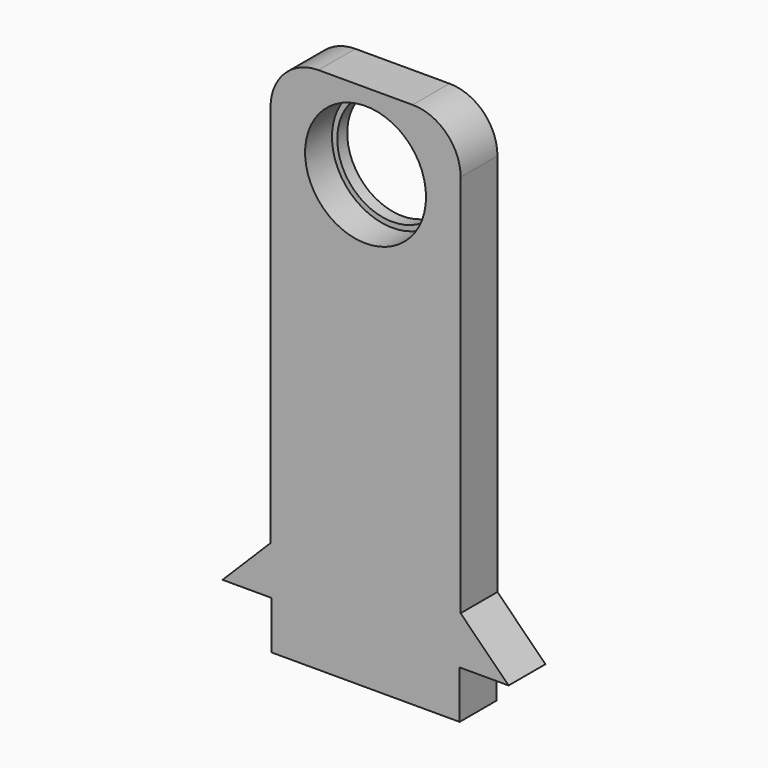
from build123d import *

# Parameters (mm, degrees)
F0_W      = 19.8
F0_H      = 55
F1_DEPTH  = 4.8
F2_R      = 5.75
F3_DEPTH  = 4.8
F4_R      = 6.3
F5_DEPTH  = 3.5
F6_W      = 4.8
F6_H      = 5
F7_DEPTH  = 5
F8_SIZE   = 4.99999
F9_W      = 4.8
F9_H      = 5
F10_DEPTH = 5
F11_SIZE  = 4.99999
F12_R     = 5
F13_DEPTH = 0.1
F14_DEPTH = 0.1


# Not quite as in the source:
# - a fillet or chamfer is up to 0.001 mm smaller than in the source, because OpenCascade refuses the exact size


with BuildPart() as f1:
    # F0 (on Front) → F1 (new body)
    with BuildSketch(Plane.XZ):
        with Locations((-0.9316042997, 16.8101646874)):
            Rectangle(F0_W, F0_H)
    extrude(amount=F1_DEPTH)

    # F2 (on face) → F3 (cut, through all)
    with BuildSketch(Plane.XZ.offset(4.8)):
        with Locations((-0.9316042997, 36.3101646874)):
            Circle(F2_R)
    extrude(amount=-F3_DEPTH, mode=Mode.SUBTRACT)

    # F4 (on face) → F5 (cut)
    with BuildSketch(Plane.XZ.offset(4.8)):
        with Locations((-0.9316042997, 36.3101646874)):
            Circle(F4_R)
    extrude(amount=-F5_DEPTH, mode=Mode.SUBTRACT)

    # F6 (on face) → F7 (join)
    with BuildSketch(Plane(origin=(-10.8316042997, 0, 0), x_dir=(0, -1, 0), z_dir=(-1, 0, 0))):
        with Locations((2.4, -3.1898353126)):
            Rectangle(F6_W, F6_H)
    extrude(amount=F7_DEPTH)

    # F8 (size 5 in the source; OpenCascade refuses exactly that, so slightly less here)
    f8_edges = [f1.edges().sort_by_distance(p)[0] for p in [
        (-15.831604, -2.4, -0.689835),
    ]]
    chamfer(f8_edges, length=F8_SIZE)

    # F9 (on face) → F10 (join)
    with BuildSketch(Plane.YZ.offset(8.9683957003)):
        with Locations((-2.4, -3.1898353126)):
            Rectangle(F9_W, F9_H)
    extrude(amount=F10_DEPTH)

    # F11 (size 5 in the source; OpenCascade refuses exactly that, so slightly less here)
    f11_edges = [f1.edges().sort_by_distance(p)[0] for p in [
        (13.968396, -2.4, -0.689835),
    ]]
    chamfer(f11_edges, length=F11_SIZE)

    # F12
    f12_edges = [f1.edges().sort_by_distance(p)[0] for p in [
        (-10.831604, -2.4, 44.310165),
        (8.968396, -2.4, 44.310165),
    ]]
    fillet(f12_edges, radius=F12_R)

    # F13 (cut): a face of the model
    f13_faces = [f1.faces().sort_by_distance(p)[0] for p in [
        (-10.8316042997, -2.4, -8.1898353126),
    ]]
    extrude(f13_faces, amount=-F13_DEPTH, mode=Mode.SUBTRACT)

    # F14 (cut): a face of the model
    f14_faces = [f1.faces().sort_by_distance(p)[0] for p in [
        (8.9683957003, -2.4, -8.1898353126),
    ]]
    extrude(f14_faces, amount=-F14_DEPTH, mode=Mode.SUBTRACT)


solid = f1.part
